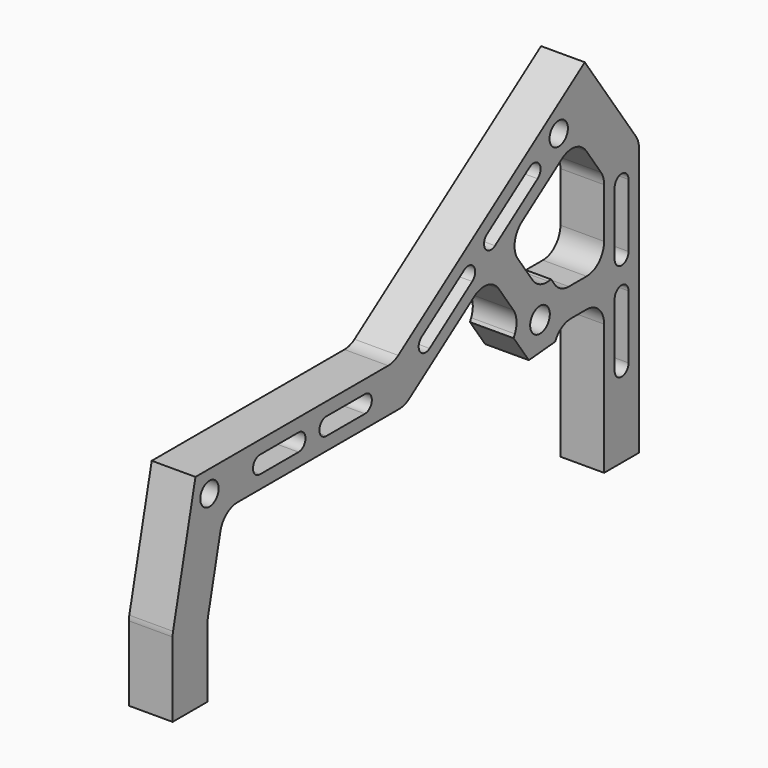
from build123d import *

# Parameters (mm, degrees)
F1_DEPTH     = 70
F2_R         = 1.685
F2_R_2       = 1.575
F3_DEPTH     = 25
F4_R         = 1.2
F5_DEPTH     = 6
F6_T1_DEPTH  = 6
F6_T6_DEPTH  = 6
F6_T8_DEPTH  = 10.7294818332
F6_T10_DEPTH = 7.6661885506


# Not quite as in the source:
# - a fillet or chamfer that OpenCascade refuses, or shapes differently, is made with other operations: its cross-section is extruded or revolved along the edge and cut away or added
# - a feature names something its author has since deleted; it is built from what else it names


with BuildPart() as f1:
    # F0 (on Top) → F1 (new body)
    with BuildSketch(Plane.XY):
        Polygon((20, 40), (14, 40), (14, 0), (14, -40), (20, -40), (20, 0), align=None)
    extrude(amount=F1_DEPTH)

    # F2 (on face) → F3 (cut)
    with BuildSketch(Plane(origin=(14, 0, 0), x_dir=(0, -1, 0), z_dir=(-1, 0, 0))):
        Polygon((-30.6819530985, 50.943057454), (2.084128673, 28), (36.084128673, 28), (40, 10.5910085265), (40, 70), (-40, 70), (-40, 37.635507345), align=None)
        Polygon((-34, 20.9578964859), (-34, 0), (34, 0), (34, 9.9245331063), (31.2838188449, 22), (0.1923359398, 22), (-14.1830926793, 32.0657834841), (-19.4291743712, 24.5736023727), (-18.4917532979, 22.5632963938), (-21.0886368482, 18.8545623277), (-25.5989365404, 19.2491624199), (-26.3957323212, 20.9578964859), align=None)
        Polygon((-34, 24.9578964859), (-26.3882395651, 24.9578964859), (-24.9154691321, 27.0612306442), (-22.7057825483, 26.8679081181), (-17.4597008565, 34.3600892295), (-29.2084994509, 42.5866865702), (-34, 35.7437146117), align=None)
        with Locations((-23.0020529902, 22.9578964859)):
            Circle(F2_R)
        with Locations((-26.2109216504, 44.1500837642)):
            Circle(F2_R_2)
        with Locations((33.683973759, 25)):
            Circle(F2_R_2)
        with BuildLine():
            Line((13.6397417612, 26.190625), (7.0209917612, 26.190625))
            ThreePointArc((7.0209917612, 26.190625), (7.8628907726, 25.8418990114), (8.2116167612, 25))
            ThreePointArc((8.2116167612, 25), (7.8628907726, 24.1581009886), (7.0209917612, 23.809375))
            Line((7.0209917612, 23.809375), (13.6397417612, 23.809375))
            ThreePointArc((13.6397417612, 23.809375), (12.4491167612, 25), (13.6397417612, 26.190625))
        make_face()
        with BuildLine():
            ThreePointArc((8.2116167612, 25), (7.8628907726, 25.8418990114), (7.0209917612, 26.190625))
            ThreePointArc((7.0209917612, 26.190625), (5.8303667612, 25), (7.0209917612, 23.809375))
            ThreePointArc((7.0209917612, 23.809375), (7.8628907726, 24.1581009886), (8.2116167612, 25))
        make_face()
        with BuildLine():
            ThreePointArc((14.8303667612, 25), (14.4816407726, 25.8418990114), (13.6397417612, 26.190625))
            ThreePointArc((13.6397417612, 26.190625), (12.4491167612, 25), (13.6397417612, 23.809375))
            ThreePointArc((13.6397417612, 23.809375), (14.4816407726, 24.1581009886), (14.8303667612, 25))
        make_face()
        with BuildLine():
            ThreePointArc((25.0209917612, 23.809375), (25.8628907726, 24.1581009886), (26.2116167612, 25))
            ThreePointArc((26.2116167612, 25), (25.8628907726, 25.8418990114), (25.0209917612, 26.190625))
            ThreePointArc((25.0209917612, 26.190625), (23.8303667612, 25), (25.0209917612, 23.809375))
        make_face()
        with BuildLine():
            ThreePointArc((25.0209917612, 23.809375), (23.8303667612, 25), (25.0209917612, 26.190625))
            Line((25.0209917612, 26.190625), (18.4022417612, 26.190625))
            ThreePointArc((18.4022417612, 26.190625), (19.2441407726, 25.8418990114), (19.5928667612, 25))
            ThreePointArc((19.5928667612, 25), (19.2441407726, 24.1581009886), (18.4022417612, 23.809375))
            Line((18.4022417612, 23.809375), (25.0209917612, 23.809375))
        make_face()
        with BuildLine():
            ThreePointArc((19.5928667612, 25), (19.2441407726, 25.8418990114), (18.4022417612, 26.190625))
            ThreePointArc((18.4022417612, 26.190625), (17.2116167612, 25), (18.4022417612, 23.809375))
            ThreePointArc((18.4022417612, 23.809375), (19.2441407726, 24.1581009886), (19.5928667612, 25))
        make_face()
        with BuildLine():
            ThreePointArc((-38.190625, 33.7249029726), (-37, 32.5342779726), (-35.809375, 33.7249029726))
            ThreePointArc((-35.809375, 33.7249029726), (-37, 34.9155279726), (-38.190625, 33.7249029726))
        make_face()
        with BuildLine():
            Line((-35.809375, 25.0294377416), (-35.809375, 33.7249029726))
            ThreePointArc((-35.809375, 33.7249029726), (-37, 32.5342779726), (-38.190625, 33.7249029726))
            Line((-38.190625, 33.7249029726), (-38.190625, 25.0294377416))
            ThreePointArc((-38.190625, 25.0294377416), (-37, 26.2200627416), (-35.809375, 25.0294377416))
        make_face()
        with BuildLine():
            ThreePointArc((-38.190625, 25.0294377416), (-37, 23.8388127416), (-35.809375, 25.0294377416))
            ThreePointArc((-35.809375, 25.0294377416), (-37, 26.2200627416), (-38.190625, 25.0294377416))
        make_face()
        with BuildLine():
            ThreePointArc((-38.190625, 11.5714725107), (-37, 10.3808475107), (-35.809375, 11.5714725107))
            ThreePointArc((-35.809375, 11.5714725107), (-37, 12.7620975107), (-38.190625, 11.5714725107))
        make_face()
        with BuildLine():
            ThreePointArc((-38.190625, 11.5714725107), (-37, 12.7620975107), (-35.809375, 11.5714725107))
            Line((-35.809375, 11.5714725107), (-35.809375, 20.2669377416))
            ThreePointArc((-35.809375, 20.2669377416), (-37, 19.0763127416), (-38.190625, 20.2669377416))
            Line((-38.190625, 20.2669377416), (-38.190625, 11.5714725107))
        make_face()
        with BuildLine():
            ThreePointArc((-38.190625, 20.2669377416), (-37, 19.0763127416), (-35.809375, 20.2669377416))
            ThreePointArc((-35.809375, 20.2669377416), (-37, 21.4575627416), (-38.190625, 20.2669377416))
        make_face()
        with BuildLine():
            ThreePointArc((-20.7184760846, 41.137916576), (-21.359331642, 40.0818193028), (-22.5920155292, 40.1626136733))
            Line((-22.5920155292, 40.1626136733), (-15.2808470158, 35.0432783671))
            ThreePointArc((-15.2808470158, 35.0432783671), (-15.573235474, 36.7014957144), (-13.9150181268, 36.9938841726))
            Line((-13.9150181268, 36.9938841726), (-21.2261866401, 42.1132194788))
            ThreePointArc((-21.2261866401, 42.1132194788), (-20.8530038114, 41.6876860187), (-20.7184760846, 41.137916576))
        make_face()
        with BuildLine():
            ThreePointArc((-21.2261866401, 42.1132194788), (-22.8844039874, 41.8208310206), (-22.5920155292, 40.1626136733))
            ThreePointArc((-22.5920155292, 40.1626136733), (-21.359331642, 40.0818193028), (-20.7184760846, 41.137916576))
            ThreePointArc((-20.7184760846, 41.137916576), (-20.8530038114, 41.6876860187), (-21.2261866401, 42.1132194788))
        make_face()
        with BuildLine():
            ThreePointArc((-13.9150181268, 36.9938841726), (-15.573235474, 36.7014957144), (-15.2808470158, 35.0432783671))
            ThreePointArc((-15.2808470158, 35.0432783671), (-14.0481631287, 34.9624839966), (-13.4073075713, 36.0185812699))
            ThreePointArc((-13.4073075713, 36.0185812699), (-13.541835298, 36.5683507125), (-13.9150181268, 36.9938841726))
        make_face()
        with BuildLine():
            ThreePointArc((-4.0684668916, 27.1922852829), (-2.8357830044, 27.1114909123), (-2.194927447, 28.1675881856))
            ThreePointArc((-2.194927447, 28.1675881856), (-2.3294551738, 28.7173576282), (-2.7026380025, 29.1428910883))
            ThreePointArc((-2.7026380025, 29.1428910883), (-4.3608553498, 28.8505026301), (-4.0684668916, 27.1922852829))
        make_face()
        with BuildLine():
            ThreePointArc((-4.0684668916, 27.1922852829), (-4.3608553498, 28.8505026301), (-2.7026380025, 29.1428910883))
            Line((-2.7026380025, 29.1428910883), (-10.0138065158, 34.2622263945))
            ThreePointArc((-10.0138065158, 34.2622263945), (-9.6406236871, 33.8366929344), (-9.5060959604, 33.2869234917))
            ThreePointArc((-9.5060959604, 33.2869234917), (-10.1469515177, 32.2308262185), (-11.3796354049, 32.311620589))
            Line((-11.3796354049, 32.311620589), (-4.0684668916, 27.1922852829))
        make_face()
        with BuildLine():
            ThreePointArc((-9.5060959604, 33.2869234917), (-9.6406236871, 33.8366929344), (-10.0138065158, 34.2622263945))
            ThreePointArc((-10.0138065158, 34.2622263945), (-11.6720238631, 33.9698379363), (-11.3796354049, 32.311620589))
            ThreePointArc((-11.3796354049, 32.311620589), (-10.1469515177, 32.2308262185), (-9.5060959604, 33.2869234917))
        make_face()
    extrude(amount=-F3_DEPTH, mode=Mode.SUBTRACT)

    # F4 (on face) → F5 (cut)
    with BuildSketch(Plane.XY):
        with Locations((17, 37)):
            Circle(F4_R)
        with Locations((17, -37)):
            Circle(F4_R)
    extrude(amount=F5_DEPTH, mode=Mode.SUBTRACT)

    # F6: fillet of radius 3 on 16 edges, made by hand

    # F6_s2 → F6_t1 (join)
    with BuildSketch(Plane.YZ.offset(14)):
        with BuildLine():
            ThreePointArc((21.7123190185, 28.286721078), (22.9019203662, 27.2885270259), (24.4312423796, 27.0188662927))
            Line((24.4312423796, 27.0188662927), (22.7057825483, 26.8679081181))
            Line((22.7057825483, 26.8679081181), (21.7123190185, 28.286721078))
        make_face()
        with BuildLine():
            ThreePointArc((25.4924845839, 26.2371671769), (26.564694877, 25.2968639864), (27.9499407167, 24.9578964859))
            Line((27.9499407167, 24.9578964859), (26.3882395651, 24.9578964859))
            Line((26.3882395651, 24.9578964859), (25.4924845839, 26.2371671769))
        make_face()
        with BuildLine():
            ThreePointArc((34, 27.9578964859), (33.1213203436, 25.8365761424), (31, 24.9578964859))
            Line((31, 24.9578964859), (34, 24.9578964859))
            Line((34, 24.9578964859), (34, 27.9578964859))
        make_face()
        with BuildLine():
            ThreePointArc((34, 34.7978182451), (33.8611508522, 35.6999356436), (33.4574561329, 36.5185475541))
            Line((33.4574561329, 36.5185475541), (34, 35.7437146117))
            Line((34, 35.7437146117), (34, 34.7978182451))
        make_face()
        with BuildLine():
            ThreePointArc((30.92922876, 40.1292304373), (28.9927171601, 41.3629243873), (26.751043318, 40.8659572611))
            Line((26.751043318, 40.8659572611), (29.2084994509, 42.5866865702))
            Line((29.2084994509, 42.5866865702), (30.92922876, 40.1292304373))
        make_face()
        with BuildLine():
            ThreePointArc((19.9171569894, 36.0808185386), (18.6834630394, 34.1443069387), (19.1804301656, 31.9026330966))
            Line((19.1804301656, 31.9026330966), (17.4597008565, 34.3600892295))
            Line((17.4597008565, 34.3600892295), (19.9171569894, 36.0808185386))
        make_face()
        with BuildLine():
            ThreePointArc((15.9038219884, 29.6083273512), (13.9673103885, 30.8420213012), (11.7256365465, 30.345054175))
            Line((11.7256365465, 30.345054175), (14.1830926793, 32.0657834841))
            Line((14.1830926793, 32.0657834841), (15.9038219884, 29.6083273512))
        make_face()
        with BuildLine():
            ThreePointArc((18.6971780696, 23.0038312383), (18.9668388028, 24.5331532517), (18.4357108414, 25.9924153326))
            Line((18.4357108414, 25.9924153326), (19.4291743712, 24.5736023727))
            Line((19.4291743712, 24.5736023727), (18.6971780696, 23.0038312383))
        make_face()
        with BuildLine():
            ThreePointArc((34, 17.9578964859), (33.1213203436, 20.0792168295), (31, 20.9578964859))
            Line((31, 20.9578964859), (34, 20.9578964859))
            Line((34, 20.9578964859), (34, 17.9578964859))
        make_face()
        with BuildLine():
            ThreePointArc((-28.8836639309, 22), (-30.7578228315, 21.3425474201), (-31.8105346625, 19.6583522769))
            Line((-31.8105346625, 19.6583522769), (-31.2838188449, 22))
            Line((-31.2838188449, 22), (-28.8836639309, 22))
        make_face()
        with BuildLine():
            ThreePointArc((-33.9268707316, 10.2496476731), (-33.9816616336, 9.9224960945), (-34, 9.5912953961))
            Line((-34, 9.5912953961), (-34, 9.9245331063))
            Line((-34, 9.9245331063), (-33.9268707316, 10.2496476731))
        make_face()
        with BuildLine():
            ThreePointArc((-3.0300250397, 28), (-2.1279076412, 28.1388491478), (-1.3092957306, 28.5425438671))
            Line((-1.3092957306, 28.5425438671), (-2.084128673, 28))
            Line((-2.084128673, 28), (-3.0300250397, 28))
        make_face()
    extrude(amount=F6_T1_DEPTH)


with BuildPart() as f6_tool4:
    # F6_s5 → F6_t6 (new body)
    with BuildSketch(Plane.YZ.offset(14)):
        with BuildLine():
            ThreePointArc((28.3069431036, 20.9578964859), (26.6950442786, 20.4880708234), (25.5880197425, 19.2257512711))
            Line((25.5880197425, 19.2257512711), (26.3957323212, 20.9578964859))
            Line((26.3957323212, 20.9578964859), (28.3069431036, 20.9578964859))
        make_face()
    extrude(amount=F6_T6_DEPTH)

    split(bisect_by=Plane(origin=(0, -1.4768383046, 16.8803390647), x_dir=(1, 0, 0), z_dir=(0, -0.0871557427, 0.9961946981)), keep=Keep.TOP)


with BuildPart() as f1_1:
    add(f1.part)

    # F6_t3: union F6_tool4
    add(f6_tool4.part)

    # F6_s9 → F6_t8 (cut)
    with BuildSketch(Plane.YZ.offset(11.6352590834)):
        with BuildLine():
            ThreePointArc((40, 36.6896109783), (39.8611508522, 37.5917283768), (39.4574561329, 38.4103402874))
            Line((39.4574561329, 38.4103402874), (40, 37.635507345))
            Line((40, 37.635507345), (40, 36.6896109783))
        make_face()
        with BuildLine():
            ThreePointArc((-1.1382323064, 22), (-0.2361149079, 22.1388491478), (0.5824970027, 22.5425438671))
            Line((0.5824970027, 22.5425438671), (-0.1923359398, 22))
            Line((-0.1923359398, 22), (-1.1382323064, 22))
        make_face()
    extrude(amount=F6_T8_DEPTH, mode=Mode.SUBTRACT)

    # F6_s11 → F6_t10 (cut)
    with BuildSketch(Plane.YZ.offset(13.1669057247)):
        with BuildLine():
            ThreePointArc((-39.9268707316, 10.9161230933), (-39.9816616336, 10.5889715148), (-40, 10.2577708164))
            Line((-40, 10.2577708164), (-40, 10.5910085265))
            Line((-40, 10.5910085265), (-39.9268707316, 10.9161230933))
        make_face()
    extrude(amount=F6_T10_DEPTH, mode=Mode.SUBTRACT)


solid = f1_1.part
